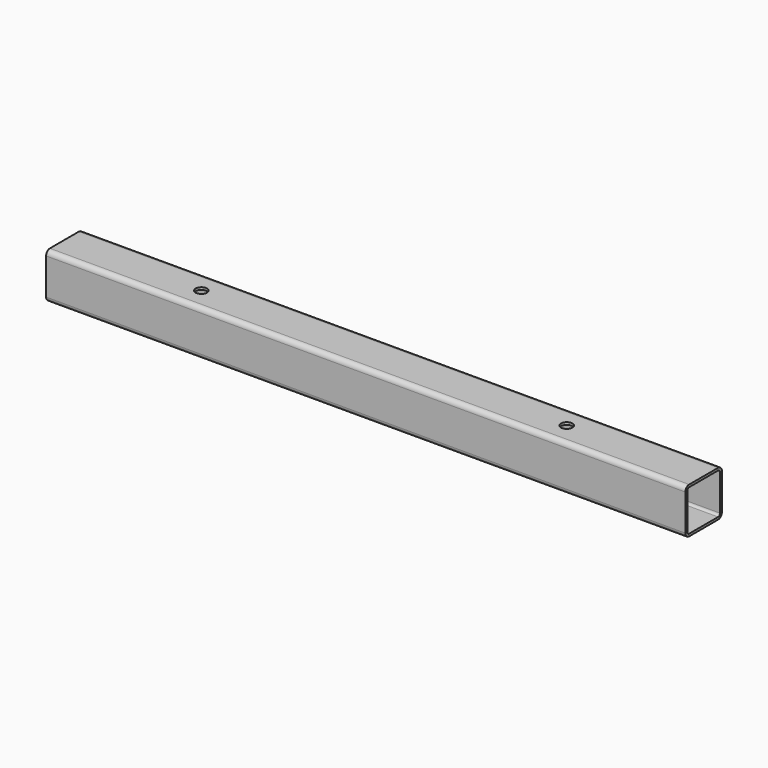
from build123d import *

# Parameters (mm, degrees)
F2_DEPTH = 444.5
F3_ANGLE = 90
F5_D     = 7.9375


# Not quite as in the source:
# - a variable given as a bare number and used for a length is read in inches; the dataset says mm whatever the document's units were


with BuildPart() as f2:
    # F0 (on Top) → F2 (new body)
    with BuildSketch(Plane.XY):
        with BuildLine():
            Line((-12.573, -15.875), (12.573, -15.875))
            ThreePointArc((12.573, -15.875), (14.9078665915, -14.9078665915), (15.875, -12.573))
            Line((15.875, -12.573), (15.875, 12.573))
            ThreePointArc((15.875, 12.573), (14.9078665915, 14.9078665915), (12.573, 15.875))
            Line((12.573, 15.875), (-12.573, 15.875))
            ThreePointArc((-12.573, 15.875), (-14.9078665915, 14.9078665915), (-15.875, 12.573))
            Line((-15.875, 12.573), (-15.875, -12.573))
            ThreePointArc((-15.875, -12.573), (-14.9078665915, -14.9078665915), (-12.573, -15.875))
        make_face()
        with BuildLine():
            Line((-12.573, 14.224), (12.573, 14.224))
            ThreePointArc((12.573, 14.224), (13.7404332957, 13.7404332957), (14.224, 12.573))
            Line((14.224, 12.573), (14.224, -12.573))
            ThreePointArc((14.224, -12.573), (13.7404332957, -13.7404332957), (12.573, -14.224))
            Line((12.573, -14.224), (-12.573, -14.224))
            ThreePointArc((-12.573, -14.224), (-13.7404332957, -13.7404332957), (-14.224, -12.573))
            Line((-14.224, -12.573), (-14.224, 12.573))
            ThreePointArc((-14.224, 12.573), (-13.7404332957, 13.7404332957), (-12.573, 14.224))
        make_face(mode=Mode.SUBTRACT)
    extrude(amount=F2_DEPTH)


with BuildPart() as f2_1:
    # F3: moved
    add(f2.part.rotate(Axis((-15.875, 0, 444.5), (0, 1, 0)), F3_ANGLE))

    # F5 (through all)
    with Locations(Plane.XY.offset(444.5)):
        with Locations((-365.125, 0), (-111.125, 0)):
            Hole(F5_D / 2)


solid = f2_1.part
